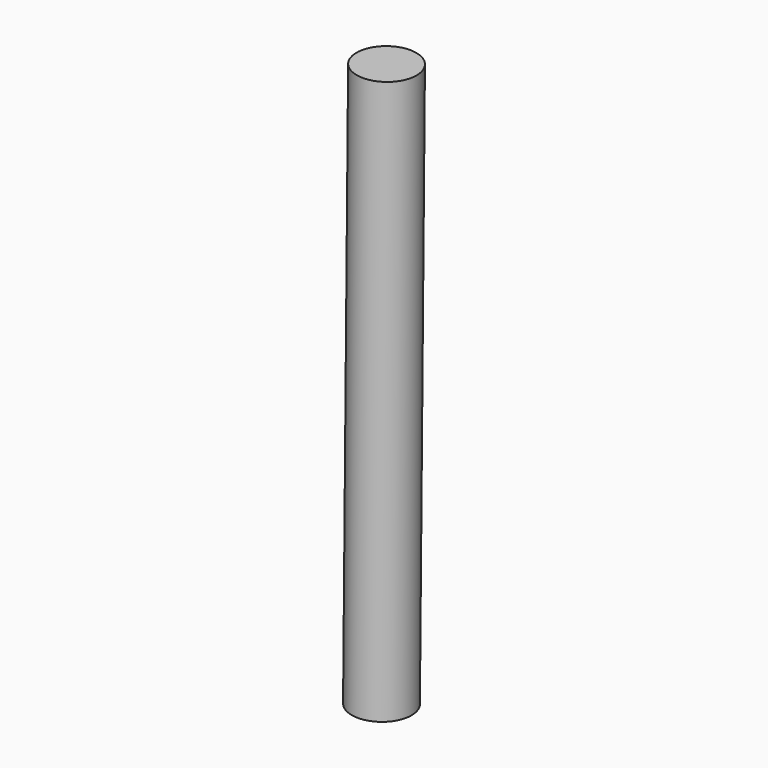
from build123d import *

# Parameters (mm, degrees)
F2_R = 50.8


with BuildPart() as f3:
    # F3: sweep along a path in F0
    with BuildLine(Plane.XZ) as f3_path:
        Line((161.1521043367, 73.1248049508), (152.6, -882.7))
    # F2 (on face) → F3 (sweep)
    with BuildSketch(Plane(origin=(-3.608930889, 0, -403.3516813269), x_dir=(0.9999599748, 0, -0.0089469974), z_dir=(-0.0089469974, 0, -0.9999599748))):
        with Locations((160.4914067552, 0)):
            Circle(F2_R)
    sweep(path=f3_path.line)


solid = f3.part
